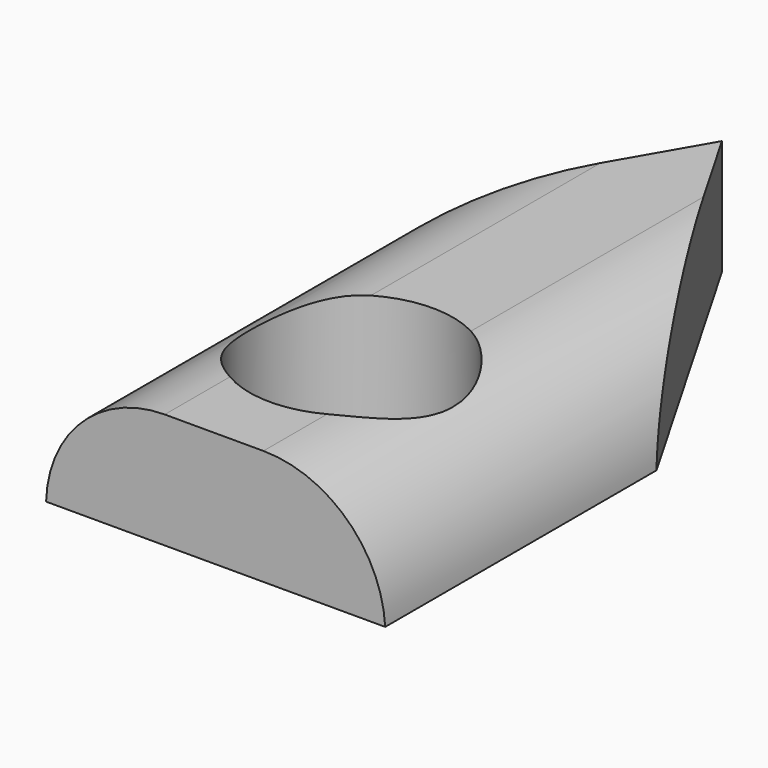
from build123d import *

# Parameters (mm, degrees)
F0_W        = 2540
F0_H        = 2540
F0_R        = 762
F1_DEPTH    = 863.6
F2_T1_DEPTH = 6983.9377403211
F3_T1_DEPTH = 7101.5479143316
F4_T        = -2.54


# Not quite as in the source:
# - a fillet or chamfer that OpenCascade refuses, or shapes differently, is made with other operations: its cross-section is extruded or revolved along the edge and cut away or added


with BuildPart() as f1:
    # F0 (on Top) → F1 (new body)
    with BuildSketch(Plane.XY):
        Rectangle(F0_W, F0_H)
        Circle(F0_R, mode=Mode.SUBTRACT)
        Polygon((0, 3469.7045256125), (-1270, 1270), (1270, 1270), align=None)
    extrude(amount=F1_DEPTH)

    # F2: fillet of radius 889.154855022 on 1 edges, made by hand

    # F2_s2 → F2_t1 (cut)
    with BuildSketch(Plane.XZ.offset(-3491.9688701606)):
        with BuildLine():
            ThreePointArc((-1270, 0), (-1000.8390059169, 612.1435766922), (-381.2124519358, 863.6))
            Line((-381.2124519358, 863.6), (-1270, 863.6))
            Line((-1270, 863.6), (-1270, 0))
        make_face()
    extrude(amount=F2_T1_DEPTH, mode=Mode.SUBTRACT)

    # F3: fillet of radius 913.6832648157 on 1 edges, made by hand

    # F3_s2 → F3_t1 (cut)
    with BuildSketch(Plane.XZ.offset(-3550.7739571658)):
        with BuildLine():
            ThreePointArc((1270, 0), (985.8054016289, 613.4592542868), (357.6904171337, 863.6))
            Line((357.6904171337, 863.6), (1270, 863.6))
            Line((1270, 863.6), (1270, 0))
        make_face()
    extrude(amount=F3_T1_DEPTH, mode=Mode.SUBTRACT)

    # F4
    f4_openings = [f1.faces().sort_by_distance(p)[0] for p in [
        (-1216.22603, 0, 0),
    ]]
    offset(amount=F4_T, openings=f4_openings)


solid = f1.part
